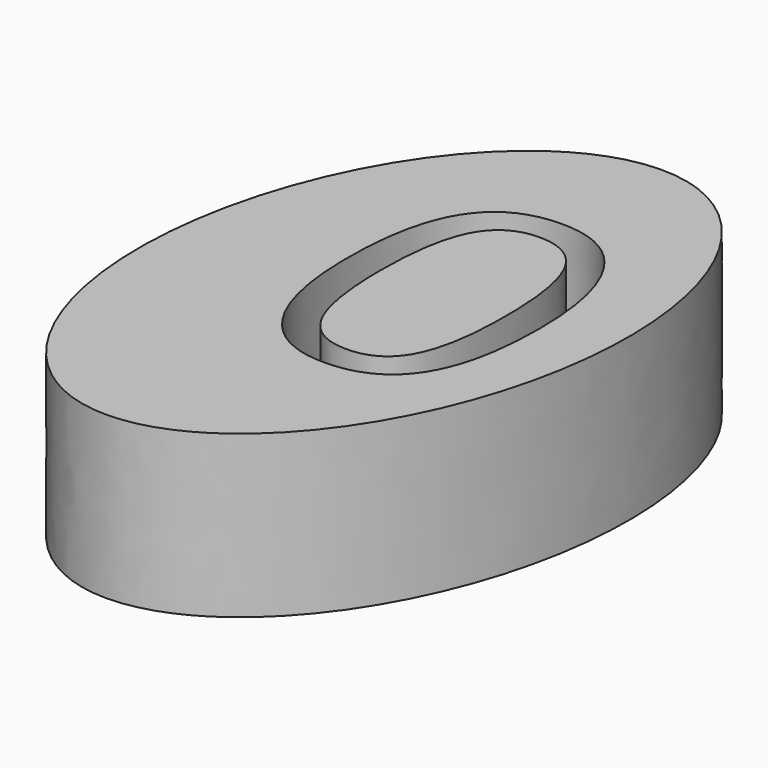
from build123d import *

# Parameters (mm, degrees)
F1_DEPTH     = 41.656
F2_TEXT_SIZE = 104.8330838482
F3_DEPTH     = 41.6570001


# Not quite as in the source:
# - Text() gives the source's letters only with a copy of the font that has no kerning and outlines rounded to 1/6400 em; it was checked with that copy


with BuildPart() as f1:
    # F0 (on Top) → F1 (new body)
    with BuildSketch(Plane.XY):
        with BuildLine():
            add(Edge.make_bspline(
                [(17.2766018659, 75.8247673512), (-65.123699313, 94.59959841), (-49.8384515224, -28.5249681461), (-34.5532037318, -151.6495347023), (32.5618496565, -47.299799205), (99.6769030448, 57.0499362923), (17.2766018659, 75.8247673512)],
                knots=[0, 0, 0, 2.0943951024, 2.0943951024, 4.1887902048, 4.1887902048, 6.2831853072, 6.2831853072, 6.2831853072], degree=2, weights=[1, 0.5, 1, 0.5, 1, 0.5, 1]))
        make_face()
    extrude(amount=F1_DEPTH)

    # F2 (on face) → F3 (cut, through all)
    with BuildSketch(Plane.XY.offset(41.656)):
        with Locations((-20.3544050455, -30.3863994777)):
            Text('0', F2_TEXT_SIZE, font='Open Sans', text_align=(TextAlign.LEFT, TextAlign.BOTTOM))
    extrude(amount=-F3_DEPTH, mode=Mode.SUBTRACT)


solid = f1.part
